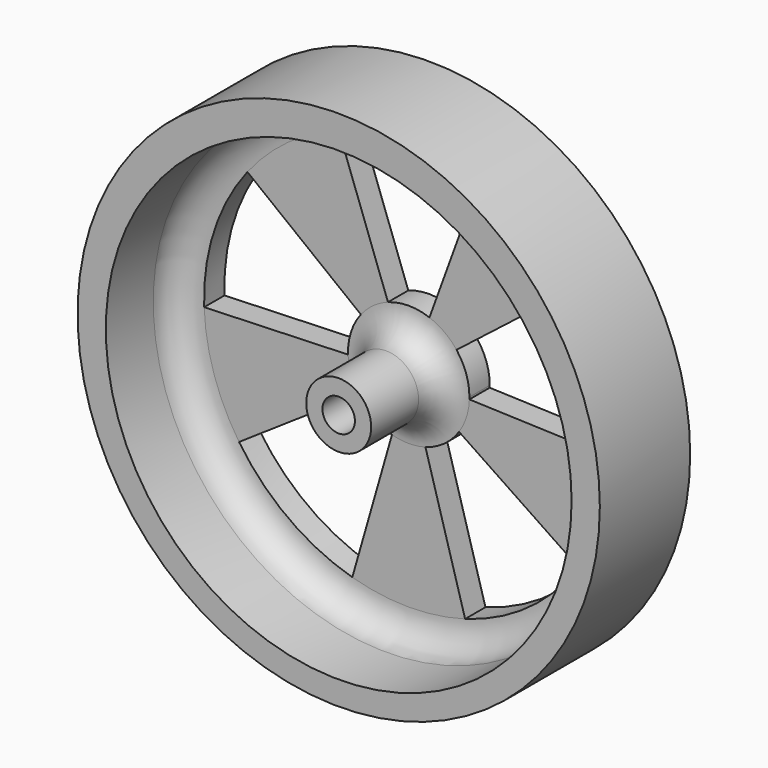
from build123d import *

# Parameters (mm, degrees)
F0_R     = 2.3
F0_R_2   = 1.15
F1_DEPTH = 8
F0_R_3   = 18.5
F0_R_4   = 16.5
F2_DEPTH = 8
F3_DEPTH = 1.8
F4_R     = 2
F6_DEPTH = 1.801


with BuildPart() as f1:
    # F0 (on Front) → F1 (new body)
    with BuildSketch(Plane.XZ):
        Circle(F0_R)
        Circle(F0_R_2, mode=Mode.SUBTRACT)
    extrude(amount=F1_DEPTH)



with BuildPart() as f2:
    # F0 (on Front) → F2 (new body)
    with BuildSketch(Plane.XZ):
        with Locations((0, 0.311320764)):
            Circle(F0_R_3)
        Circle(F0_R_4, mode=Mode.SUBTRACT)
    extrude(amount=F2_DEPTH)


with BuildPart() as f1_1:
    add(f1.part)

    add(f2.part)  # F3 merges F2
    # F0 (on Front) → F3 (join)
    with BuildSketch(Plane.XZ):
        with Locations((0, 0.311320764)):
            Circle(F0_R_3)
        Circle(F0_R_4, mode=Mode.SUBTRACT)
        Circle(F0_R_4)
        Circle(F0_R, mode=Mode.SUBTRACT)
        Circle(F0_R)
        Circle(F0_R_2, mode=Mode.SUBTRACT)
        Circle(F0_R_2)
    extrude(amount=F3_DEPTH)

    # F4
    f4_edges = [f1_1.edges().sort_by_distance(p)[0] for p in [
        (-16.5, -1.8, 0),
        (-2.3, -1.8, 0),
    ]]
    fillet(f4_edges, radius=F4_R)

    # F5 (on face) → F6 (cut, through all)
    with BuildSketch(Plane.XZ.offset(1.8)):
        with BuildLine():
            Line((1.4706866163, 4.0406782694), (4.9592920782, 13.6255430014))
            ThreePointArc((4.9592920782, 13.6255430014), (0, 14.5), (-4.9592920782, 13.6255430014))
            Line((-4.9592920782, 13.6255430014), (-1.4706866163, 4.0406782694))
            ThreePointArc((-1.4706866163, 4.0406782694), (0, 4.3), (1.4706866163, 4.0406782694))
        make_face()
        with BuildLine():
            ThreePointArc((14.4911669918, -0.5060427022), (14.4977915798, -0.2530598933), (14.5, 0))
            ThreePointArc((14.5, 0), (13.7100193462, 4.7207382396), (11.4261559273, 8.9270913922))
            Line((11.4261559273, 8.9270913922), (3.3884462405, 2.6473443439))
            ThreePointArc((3.3884462405, 2.6473443439), (4.0657298751, 1.3999430642), (4.3, 0))
            ThreePointArc((4.3, 0), (4.2993450892, -0.0750453477), (4.2973805562, -0.1500678358))
            Line((4.2973805562, -0.1500678358), (14.4911669918, -0.5060427022))
        make_face()
        with BuildLine():
            ThreePointArc((3.9967416593, -13.9382945911), (8.5228861582, -11.7307464184), (12.021044802, -8.1082971003))
            Line((12.021044802, -8.1082971003), (3.564861562, -2.4045294849))
            ThreePointArc((3.564861562, -2.4045294849), (2.5274765849, -3.4787730758), (1.18524063, -4.1334252925))
            Line((1.18524063, -4.1334252925), (3.9967416593, -13.9382945911))
        make_face()
        with BuildLine():
            ThreePointArc((-12.021044802, -8.1082971003), (-8.5228861582, -11.7307464184), (-3.9967416593, -13.9382945911))
            Line((-3.9967416593, -13.9382945911), (-1.18524063, -4.1334252925))
            ThreePointArc((-1.18524063, -4.1334252925), (-2.5274765849, -3.4787730758), (-3.564861562, -2.4045294849))
            Line((-3.564861562, -2.4045294849), (-12.021044802, -8.1082971003))
        make_face()
        with BuildLine():
            Line((-3.3884462405, 2.6473443439), (-11.4261559273, 8.9270913922))
            ThreePointArc((-11.4261559273, 8.9270913922), (-13.7903194863, 4.4807464184), (-14.4911669918, -0.5060427022))
            Line((-14.4911669918, -0.5060427022), (-4.2973805562, -0.1500678358))
            ThreePointArc((-4.2973805562, -0.1500678358), (-4.0895430201, 1.3287730758), (-3.3884462405, 2.6473443439))
        make_face()
    extrude(amount=-F6_DEPTH, mode=Mode.SUBTRACT)


solid = f1_1.part
